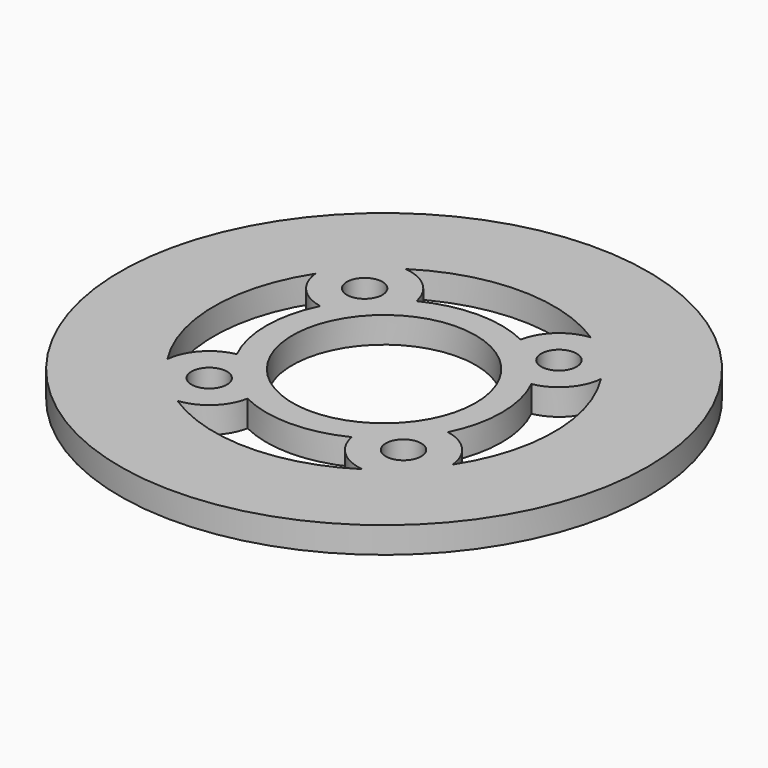
from build123d import *

# Parameters (mm, degrees)
F0_R            = 32.0294
F0_R_2          = 2.15265
F0_R_3          = 11.1125
F1_DEPTH        = 3.175
F3_DEPTH        = 3.175
F3_COPIES_COUNT = 4


# Not quite as in the source:
# - a pattern or mirror of a feature is missing from the dataset's text; its kind, count and spacing are read off the source's solid


with BuildPart() as f1:
    # F0 (on Top) → F1 (new body)
    with BuildSketch(Plane.XY):
        Circle(F0_R)
        with Locations((-11.7865861589, -11.7865861589)):
            Circle(F0_R_2, mode=Mode.SUBTRACT)
        with Locations((11.7865861589, -11.7865861589)):
            Circle(F0_R_2, mode=Mode.SUBTRACT)
        with Locations((-11.7865861589, 11.7865861589)):
            Circle(F0_R_2, mode=Mode.SUBTRACT)
        Circle(F0_R_3, mode=Mode.SUBTRACT)
        with Locations((11.7865861589, 11.7865861589)):
            Circle(F0_R_2, mode=Mode.SUBTRACT)
    extrude(amount=F1_DEPTH)

    # F2 (on face) → F3 (cut, through all)
    with BuildSketch(Plane.XY.offset(3.175)):
        with BuildLine():
            ThreePointArc((-11.229543123, 17.3148424047), (-8.0281867, 15.8788163052), (-6.3255746232, 12.8109235396))
            ThreePointArc((-6.3255746232, 12.8109235396), (0, 14.2875), (6.3255746232, 12.8109235396))
            ThreePointArc((6.3255746232, 12.8109235396), (8.0281867, 15.8788163052), (11.229543123, 17.3148424047))
            ThreePointArc((11.229543123, 17.3148424047), (0, 20.6375), (-11.229543123, 17.3148424047))
        make_face()
    f3 = extrude(amount=-F3_DEPTH, mode=Mode.SUBTRACT)

    # F3_copies: F3 ×4 about axis
    f3_copies_axis = Axis((0, 0, 0), (0, 0, 1))
    for i in range(1, F3_COPIES_COUNT):
        add(f3.rotate(f3_copies_axis, i * 360 / F3_COPIES_COUNT), mode=Mode.SUBTRACT)


solid = f1.part
